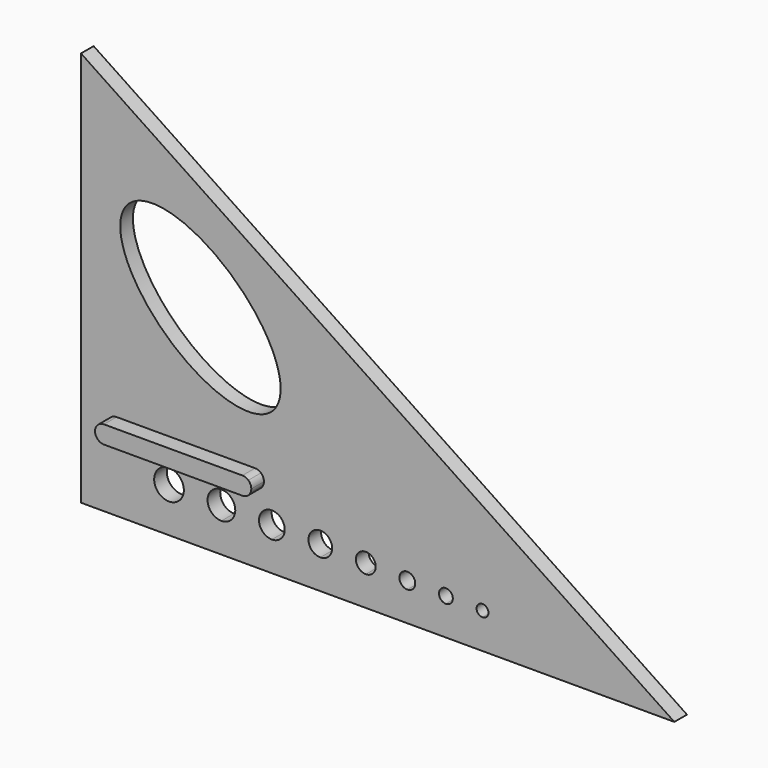
from build123d import *

# Parameters (mm, degrees)
F1_DEPTH  = 8
F3_DEPTH  = 25
F5_DEPTH  = 8
F7_DEPTH  = 25
F9_DEPTH  = 25
F11_DEPTH = 25


with BuildPart() as f1:
    # F0 (on Front) → F1 (new body)
    with BuildSketch(Plane.XZ):
        Polygon((0, 200), (0, 0), (300, 0), align=None)
    extrude(amount=F1_DEPTH)

    # F2 (on face) → F3 (cut)
    with BuildSketch(Plane.XZ.offset(8)):
        with BuildLine():
            ThreePointArc((103, 21.5), (91.9038059223, 26.0961940777), (96.5, 15))
            ThreePointArc((96.5, 15), (101.0961940777, 16.9038059223), (103, 21.5))
        make_face()
        with BuildLine():
            ThreePointArc((127, 21), (116.7573593129, 25.2426406871), (121, 15))
            ThreePointArc((121, 15), (125.2426406871, 16.7573593129), (127, 21))
        make_face()
        with BuildLine():
            ThreePointArc((149, 20), (140.4644660941, 23.5355339059), (144, 15))
            ThreePointArc((144, 15), (147.5355339059, 16.4644660941), (149, 20))
        make_face()
        with BuildLine():
            ThreePointArc((169, 19), (162.1715728753, 21.8284271247), (165, 15))
            ThreePointArc((165, 15), (167.8284271247, 16.1715728753), (169, 19))
        make_face()
        with BuildLine():
            ThreePointArc((188, 18.5), (182.0251262658, 20.9748737342), (184.5, 15))
            ThreePointArc((184.5, 15), (186.9748737342, 16.0251262658), (188, 18.5))
        make_face()
        with BuildLine():
            ThreePointArc((206, 18), (200.8786796564, 20.1213203436), (203, 15))
            ThreePointArc((203, 15), (205.1213203436, 15.8786796564), (206, 18))
        make_face()
    extrude(amount=-F3_DEPTH, mode=Mode.SUBTRACT)

    # F4 (on face) → F5 (join)
    with BuildSketch(Plane.XZ.offset(8)):
        with BuildLine():
            ThreePointArc((15, 42.8541019662), (13.5, 39.5), (15, 36.1458980338))
            Line((15, 36.1458980338), (15, 39.5))
            Line((15, 39.5), (15, 42.8541019662))
        make_face()
        with BuildLine():
            Line((15, 39.5), (15, 36.1458980338))
            ThreePointArc((15, 36.1458980338), (16.3943005877, 35.2962243879), (17.9999999821, 35))
            ThreePointArc((17.9999999821, 35), (21.181980509, 36.3180194783), (22.5, 39.5))
            ThreePointArc((22.5, 39.5), (21.1819805153, 42.6819805153), (18, 44))
            ThreePointArc((18, 44), (16.394300596, 43.7037756153), (15, 42.8541019662))
            Line((15, 42.8541019662), (15, 39.5))
        make_face()
        with BuildLine():
            ThreePointArc((22.5, 39.5), (21.181980509, 36.3180194783), (17.9999999821, 35))
            Line((17.9999999821, 35), (88, 35))
            ThreePointArc((88, 35), (83.5, 39.5), (88, 44))
            Line((88, 44), (18, 44))
            ThreePointArc((18, 44), (21.1819805153, 42.6819805153), (22.5, 39.5))
        make_face()
        with BuildLine():
            ThreePointArc((88, 44), (83.5, 39.5), (88, 35))
            ThreePointArc((88, 35), (89.605699404, 35.2962243847), (91, 36.1458980338))
            Line((91, 36.1458980338), (91, 39.5))
            Line((91, 39.5), (91, 42.8541019662))
            ThreePointArc((91, 42.8541019662), (89.605699404, 43.7037756153), (88, 44))
        make_face()
        with BuildLine():
            Line((91, 39.5), (91, 36.1458980338))
            ThreePointArc((91, 36.1458980338), (92.1079191813, 37.6628826929), (92.5, 39.5))
            ThreePointArc((92.5, 39.5), (92.1079191813, 41.3371173071), (91, 42.8541019662))
            Line((91, 42.8541019662), (91, 39.5))
        make_face()
    extrude(amount=F5_DEPTH)

    # F6 (on face) → F7 (cut)
    with BuildSketch(Plane.XZ.offset(8)):
        with BuildLine():
            add(Edge.make_bspline(
                [(97.2316949817, 72.7356295876), (126.5063207343, 104.641683669), (56.60610112, 139.3937958045), (-13.2941184942, 174.1459079399), (27.3314753674, 107.4877417231), (67.957069229, 40.8295755063), (97.2316949817, 72.7356295876)],
                knots=[0, 0, 0, 2.0943951024, 2.0943951024, 4.1887902048, 4.1887902048, 6.2831853072, 6.2831853072, 6.2831853072], degree=2, weights=[1, 0.5, 1, 0.5, 1, 0.5, 1]))
        make_face()
    extrude(amount=-F7_DEPTH, mode=Mode.SUBTRACT)

    # F8 (on face) → F9 (cut)
    with BuildSketch(Plane.XZ.offset(8)):
        with BuildLine():
            Line((71, 21.5), (71, 15))
            ThreePointArc((71, 15), (75.7696960071, 16.876524617), (77.9821200219, 21.5))
            Line((77.9821200219, 21.5), (71, 21.5))
        make_face()
        with BuildLine():
            ThreePointArc((78, 22), (66.0502525317, 26.9497474683), (71, 15))
            Line((71, 15), (71, 21.5))
            Line((71, 21.5), (77.9821200219, 21.5))
            ThreePointArc((77.9821200219, 21.5), (77.9955285774, 21.7498402043), (78, 22))
        make_face()
    extrude(amount=-F9_DEPTH, mode=Mode.SUBTRACT)

    # F10 (on face) → F11 (cut)
    with BuildSketch(Plane.XZ.offset(8)):
        with BuildLine():
            ThreePointArc((52, 22.5), (39.1966991411, 27.8033008589), (44.5, 15))
            ThreePointArc((44.5, 15), (49.8033008589, 17.1966991411), (52, 22.5))
        make_face()
    extrude(amount=-F11_DEPTH, mode=Mode.SUBTRACT)


solid = f1.part
